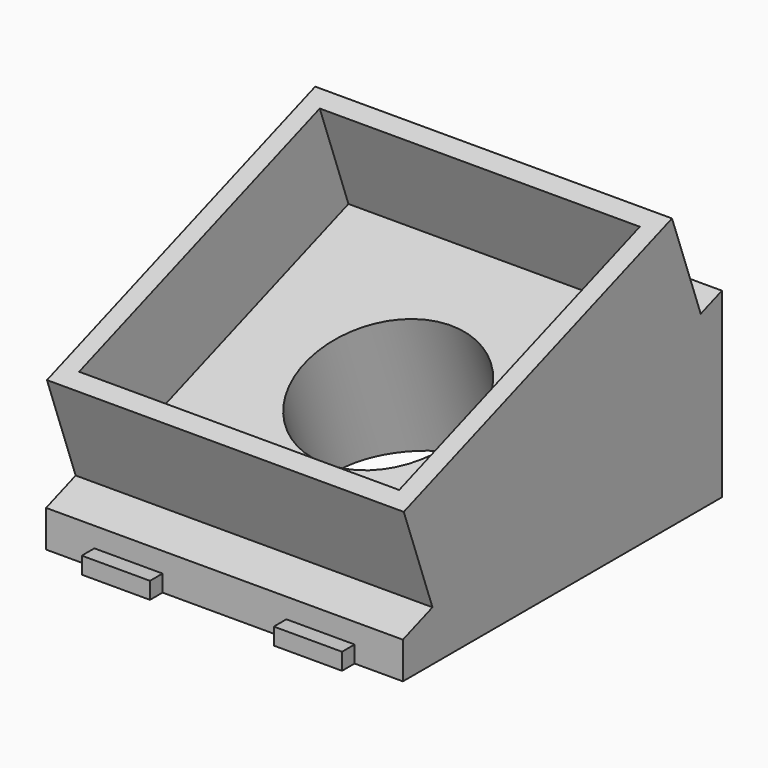
from build123d import *

# Parameters (mm, degrees)
F1_DEPTH = 1.6
F3_DEPTH = 20
F5_DEPTH = 34.001
F6_W     = 34
F6_H     = 34
F6_W_2   = 30.5
F6_H_2   = 30.5
F7_DEPTH = 10
F6_R     = 8
F8_DEPTH = 16.7997198341


# Not quite as in the source:
# - a feature names something its author has since deleted; it is built from what else it names


with BuildPart() as f1:
    # F0 (on Top) → F1 (new body)
    with BuildSketch(Plane.XY):
        Polygon((-12.4, 19), (-17, 19), (-17, -19), (-12.4, -19), (-12.4, -20.5), (-5.9, -20.5), (-5.9, -19), (5.9, -19), (5.9, -20.5), (12.4, -20.5), (12.4, -19), (17, -19), (17, 19), (12.4, 19), (12.4, 20.5), (5.9, 20.5), (5.9, 19), (-5.9, 19), (-5.9, 20.5), (-12.4, 20.5), align=None)
    extrude(amount=F1_DEPTH)

    # F2 (on face) → F3 (join)
    with BuildSketch(Plane.XY.offset(1.6)):
        Polygon((-12.4, 19), (-17, 19), (-17, -19), (-12.4, -19), (-5.9, -19), (5.9, -19), (12.4, -19), (17, -19), (17, 19), (12.4, 19), (5.9, 19), (-5.9, 19), align=None)
    extrude(amount=F3_DEPTH)

    # F4 (on face) → F5 (cut, through all)
    with BuildSketch(Plane(origin=(-17, 0, 0), x_dir=(0, -1, 0), z_dir=(-1, 0, 0))):
        Polygon((-19, 17.3308689021), (19, 3.5), (19, 21.6), (-19, 21.6), align=None)
    extrude(amount=-F5_DEPTH, mode=Mode.SUBTRACT)

    # F6 (on face) → F7 (join)
    with BuildSketch(Plane(origin=(0, -3.3474561073, 9.1970600675), x_dir=(1, 0, 0), z_dir=(0, -0.3420201433, 0.9396926208))):
        with Locations((0, 4.0929107067)):
            Rectangle(F6_W, F6_H)
        with Locations((0, 4.0929107067)):
            Rectangle(F6_W_2, F6_H_2, mode=Mode.SUBTRACT)
    extrude(amount=F7_DEPTH)

    # F6 (on face) → F8 (cut, through all)
    with BuildSketch(Plane(origin=(0, -3.3474561073, 9.1970600675), x_dir=(1, 0, 0), z_dir=(0, -0.3420201433, 0.9396926208))):
        with Locations((0, 4.0929107067)):
            Circle(F6_R)
    extrude(amount=-F8_DEPTH, mode=Mode.SUBTRACT)


solid = f1.part
